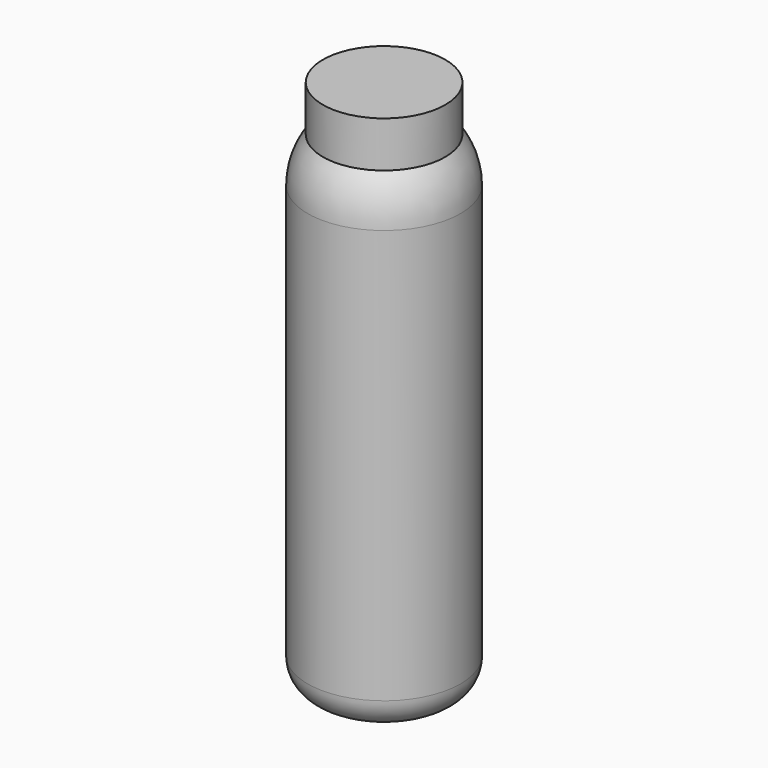
from build123d import *

# Parameters (mm, degrees)
F0_R     = 25.4
F1_DEPTH = 19.05
F2_R     = 31.75
F3_DEPTH = 203.2
F4_R     = 12.7


# Not quite as in the source:
# - a fillet or chamfer that OpenCascade refuses, or shapes differently, is made with other operations: its cross-section is extruded or revolved along the edge and cut away or added


with BuildPart() as f1:
    # F0 (on Top) → F1 (new body)
    with BuildSketch(Plane.XY):
        Circle(F0_R)
    extrude(amount=-F1_DEPTH)

    # F2 (on face) → F3 (join)
    with BuildSketch(Plane(origin=(0, 0, -19.05), x_dir=(1, 0, 0), z_dir=(0, 0, -1))):
        Circle(F2_R)
    extrude(amount=F3_DEPTH)

    # F4
    f4_edges = [f1.edges().sort_by_distance(p)[0] for p in [
        (-31.75, 0, -222.25),
    ]]
    fillet(f4_edges, radius=F4_R)

    # F5: fillet of radius 30.48 on 1 edges, made by hand

    # F5_s1 → F5_t2 (revolve, cut)
    with BuildSketch(Plane.XZ):
        with BuildLine():
            ThreePointArc((31.75, -37.6718554392), (30.1188543967, -27.8344777399), (25.4, -19.05))
            Line((25.4, -19.05), (31.75, -19.05))
            Line((31.75, -19.05), (31.75, -37.6718554392))
        make_face()
    revolve(axis=Axis((0, 0, -19.05), (0, 0, -1)), mode=Mode.SUBTRACT)


solid = f1.part
